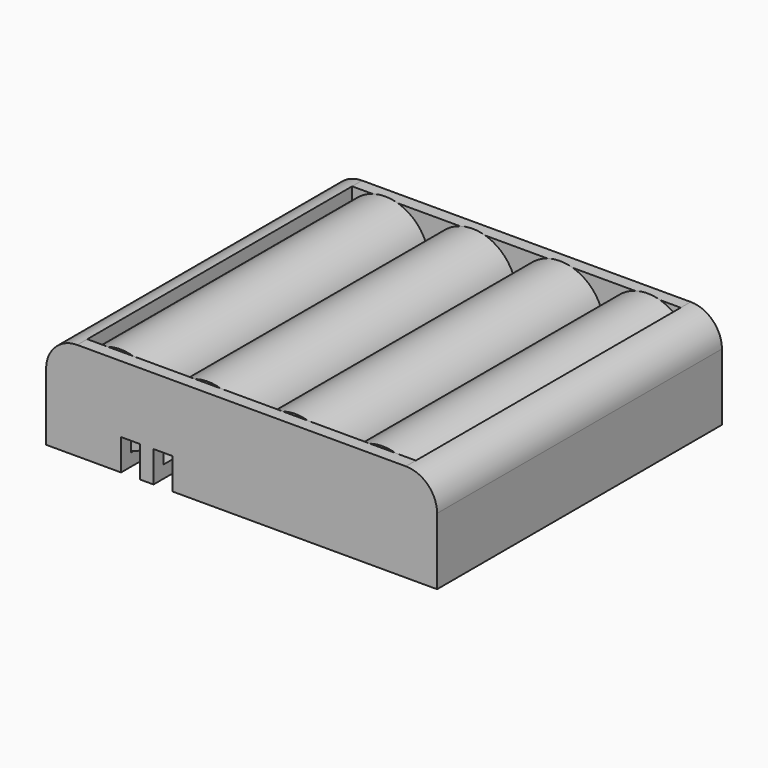
from build123d import *

# Parameters (mm, degrees)
F0_W     = 62.6
F0_H     = 57
F1_DEPTH = 15.7
F2_R     = 5
F3_T     = -2
F4_W     = 3
F4_H     = 5
F5_DEPTH = 4
F6_R     = 1.25
F7_DEPTH = 25
F9_DEPTH = 53
F8_R     = 7


# Not quite as in the source:
# - a shell that OpenCascade refuses in one call is made with other operations: the cavity is built on its own and cut out


with BuildPart() as f1:
    # F0 (on Top) → F1 (new body)
    with BuildSketch(Plane.XY):
        Rectangle(F0_W, F0_H)
    extrude(amount=F1_DEPTH)

    # F2
    f2_edges = [f1.edges().sort_by_distance(p)[0] for p in [
        (-31.3, 0, 15.7),
        (31.3, 0, 15.7),
    ]]
    fillet(f2_edges, radius=F2_R)

    # F3: a shell. OpenCascade refuses it in one call, so the cavity is built on its own and cut out:
    # the body offset inwards by the wall thickness, plus a prism from it out through each open face.
    f3_core = offset(f1.part, amount=F3_T, mode=Mode.PRIVATE)
    f3_exits = [f3_core.faces().sort_by_distance(p)[0] for p in [
        (0, 0, 13.7),
    ]]
    add(f3_core, mode=Mode.SUBTRACT)
    extrude(f3_exits, amount=-F3_T, mode=Mode.SUBTRACT)

    # F4 (on face) → F5 (cut)
    with BuildSketch(Plane.XZ.offset(28.5)):
        with Locations((-17.8, 2.5)):
            Rectangle(F4_W, F4_H)
        with Locations((-12.6, 2.5)):
            Rectangle(F4_W, F4_H)
    extrude(amount=-F5_DEPTH, mode=Mode.SUBTRACT)

    # F6 (on face) → F7 (cut)
    with BuildSketch(Plane(origin=(0, 0, 0), x_dir=(1, 0, 0), z_dir=(0, 0, -1))):
        with Locations((-22.95, 0)):
            Circle(F6_R)
        with Locations((22.95, 0)):
            Circle(F6_R)
        with Locations((-7.45, 0)):
            Circle(F6_R)
        with Locations((7.45, 0)):
            Circle(F6_R)
    extrude(amount=-F7_DEPTH, mode=Mode.SUBTRACT)


with BuildPart() as f9:
    # F8 (on face) → F9 (new body, through all)
    with BuildSketch(Plane.XZ.offset(-26.5)):
        with BuildLine():
            ThreePointArc((14, 9), (21, 2), (28, 9))
            ThreePointArc((28, 9), (21, 16), (14, 9))
        make_face()
    extrude(amount=F9_DEPTH)


with BuildPart() as f9b:
    # F8 (on face) → F9, piece 2 (new body, through all)
    with BuildSketch(Plane.XZ.offset(-26.5)):
        with Locations((-21, 9)):
            Circle(F8_R)
    extrude(amount=F9_DEPTH)


with BuildPart() as f9c:
    # F8 (on face) → F9, piece 3 (new body, through all)
    with BuildSketch(Plane.XZ.offset(-26.5)):
        with BuildLine():
            ThreePointArc((-14, 9), (-7, 2), (0, 9))
            ThreePointArc((0, 9), (-7, 16), (-14, 9))
        make_face()
    extrude(amount=F9_DEPTH)


with BuildPart() as f9d:
    # F8 (on face) → F9, piece 4 (new body, through all)
    with BuildSketch(Plane.XZ.offset(-26.5)):
        with BuildLine():
            ThreePointArc((0, 9), (7, 2), (14, 9))
            ThreePointArc((14, 9), (7, 16), (0, 9))
        make_face()
    extrude(amount=F9_DEPTH)


solid = Compound([f1.part, f9.part, f9b.part, f9c.part, f9d.part])
